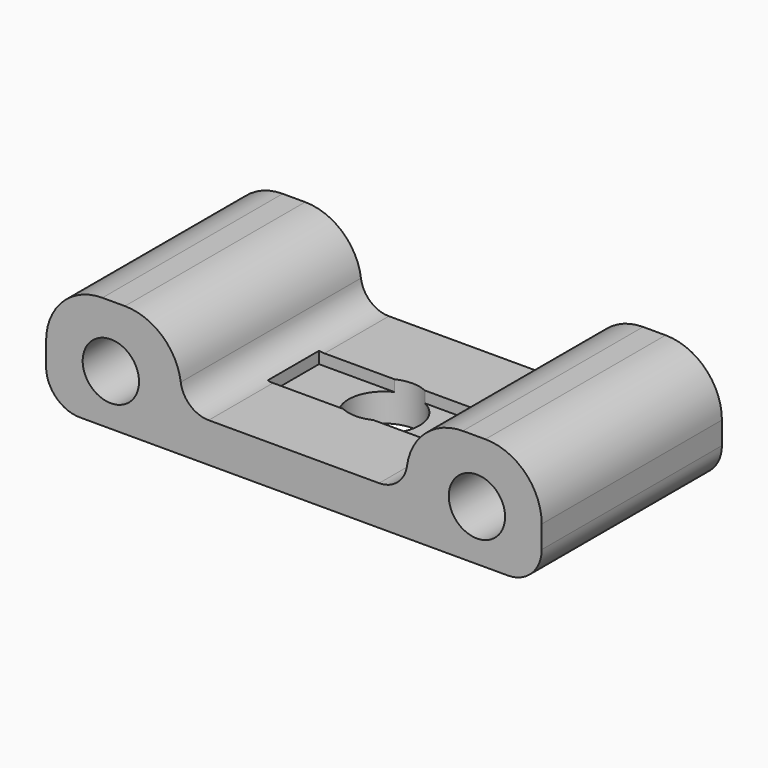
from build123d import *

# Parameters (mm, degrees)
F0_W          = 36
F0_H          = 20
F1_DEPTH      = 3.5
F3_DEPTH      = 1
F4_W          = 4
F4_H          = 20
F4_W_2        = 8
F5_DEPTH      = 10
F6_R          = 2.5
F7_DEPTH      = 20.001
F8_R          = 5
F9_R          = 3
F10_T4_DEPTH  = 20
F10_T10_DEPTH = 20
F10_T16_DEPTH = 20
F10_T23_DEPTH = 20
F10_T29_DEPTH = 20
F10_T35_DEPTH = 20
F10_T41_DEPTH = 20
F10_T47_DEPTH = 20
F10_T54_DEPTH = 20
F10_T60_DEPTH = 20


# Not quite as in the source:
# - a fillet or chamfer that OpenCascade refuses, or shapes differently, is made with other operations: its cross-section is extruded or revolved along the edge and cut away or added


with BuildPart() as f1:
    # F0 (on Top) → F1 (new body)
    with BuildSketch(Plane.XY):
        Rectangle(F0_W, F0_H)
        with BuildLine():
            ThreePointArc((3.15, 0), (0, -3.15), (-3.15, 0))
            ThreePointArc((-3.15, 0), (0, 3.15), (3.15, 0))
        make_face(mode=Mode.SUBTRACT)
    extrude(amount=F1_DEPTH)

    # F2 (on face) → F3 (cut)
    with BuildSketch(Plane.XY.offset(3.5)):
        with BuildLine():
            Line((-1.3416407865, 2.85), (-8.05, 2.85))
            Line((-8.05, 2.85), (-8.05, -2.85))
            Line((-8.05, -2.85), (-1.3416407865, -2.85))
            ThreePointArc((-1.3416407865, -2.85), (-3.15, 0), (-1.3416407865, 2.85))
        make_face()
        with BuildLine():
            Line((1.3416407865, 2.85), (-1.3416407865, 2.85))
            ThreePointArc((-1.3416407865, 2.85), (-3.15, 0), (-1.3416407865, -2.85))
            Line((-1.3416407865, -2.85), (1.3416407865, -2.85))
            ThreePointArc((1.3416407865, -2.85), (2.6597620643, -1.6876509595), (3.15, 0))
            ThreePointArc((3.15, 0), (2.6597620643, 1.6876509595), (1.3416407865, 2.85))
        make_face()
        with BuildLine():
            Line((8.05, 2.85), (1.3416407865, 2.85))
            ThreePointArc((1.3416407865, 2.85), (2.6597620643, 1.6876509595), (3.15, 0))
            ThreePointArc((3.15, 0), (2.6597620643, -1.6876509595), (1.3416407865, -2.85))
            Line((1.3416407865, -2.85), (8.05, -2.85))
            Line((8.05, -2.85), (8.05, 2.85))
        make_face()
    extrude(amount=-F3_DEPTH, mode=Mode.SUBTRACT)

    # F4 (on Top) → F5 (join)
    with BuildSketch(Plane.XY):
        with Locations((20, 0)):
            Rectangle(F4_W, F4_H)
        with Locations((14, 0)):
            Rectangle(F4_W_2, F4_H)
        with Locations((-14, 0)):
            Rectangle(F4_W_2, F4_H)
        with Locations((-20, 0)):
            Rectangle(F4_W, F4_H)
    extrude(amount=F5_DEPTH)

    # F6 (on face) → F7 (cut, through all)
    with BuildSketch(Plane.XZ.offset(10)):
        with Locations((-16.25, 4.5)):
            Circle(F6_R)
        with BuildLine():
            ThreePointArc((18.75, 4.5), (16.25, 7), (13.75, 4.5))
            ThreePointArc((13.75, 4.5), (16.25, 2), (18.75, 4.5))
        make_face()
    extrude(amount=-F7_DEPTH, mode=Mode.SUBTRACT)

    # F8
    f8_edges = [f1.edges().sort_by_distance(p)[0] for p in [
        (-22, 0, 10),
        (-10, 0, 10),
        (10, 0, 10),
        (22, 0, 10),
    ]]
    fillet(f8_edges, radius=F8_R)

    # F9
    f9_edges = [f1.edges().sort_by_distance(p)[0] for p in [
        (-22, 0, 0),
        (22, 0, 0),
    ]]
    fillet(f9_edges, radius=F9_R)

    # F10: fillet of radius 2.5 on 2 edges, made by hand


with BuildPart() as f10_tool2:
    # F10_s3 → F10_t4 (new body)
    with BuildSketch(Plane.XZ.offset(10)):
        with BuildLine():
            ThreePointArc((10.0446437509, 5.6666666667), (9.2126670979, 4.1180683682), (7.5669656263, 3.5))
            Line((7.5669656263, 3.5), (7.5669656263, 3.25))
            Line((7.5669656263, 3.25), (10, 3.25))
            Line((10, 3.25), (10.25, 3.5))
            ThreePointArc((10.25, 3.5), (10.25, 5), (10.2924115633, 5.6333333333))
            Line((10.2924115633, 5.6333333333), (10.0446437509, 5.6666666667))
        make_face()
    extrude(amount=-F10_T4_DEPTH)

    split(bisect_by=Plane.YZ.offset(8.05), keep=Keep.TOP)

    split(bisect_by=Plane.XZ.offset(2.85), keep=Keep.TOP)


with BuildPart() as f1_1:
    add(f1.part)

    # F10_t1: union F10_tool2
    add(f10_tool2.part)


with BuildPart() as f10_tool8:
    # F10_s9 → F10_t10 (new body)
    with BuildSketch(Plane.XZ.offset(10)):
        with BuildLine():
            ThreePointArc((10.0446437509, 5.6666666667), (9.2126670979, 4.1180683682), (7.5669656263, 3.5))
            Line((7.5669656263, 3.5), (7.5669656263, 3.25))
            Line((7.5669656263, 3.25), (10, 3.25))
            Line((10, 3.25), (10.25, 3.5))
            ThreePointArc((10.25, 3.5), (10.25, 5), (10.2924115633, 5.6333333333))
            Line((10.2924115633, 5.6333333333), (10.0446437509, 5.6666666667))
        make_face()
    extrude(amount=-F10_T10_DEPTH)

    split(bisect_by=Plane.YZ.offset(8.05), keep=Keep.BOTTOM)

    split(bisect_by=Plane.XZ.offset(2.85), keep=Keep.TOP)


with BuildPart() as f1_2:
    add(f1_1.part)

    # F10_t7: union F10_tool8
    add(f10_tool8.part)


with BuildPart() as f10_tool14:
    # F10_s15 → F10_t16 (new body)
    with BuildSketch(Plane.XZ.offset(10)):
        with BuildLine():
            ThreePointArc((10.0446437509, 5.6666666667), (9.2126670979, 4.1180683682), (7.5669656263, 3.5))
            Line((7.5669656263, 3.5), (7.5669656263, 3.25))
            Line((7.5669656263, 3.25), (10, 3.25))
            Line((10, 3.25), (10.25, 3.5))
            ThreePointArc((10.25, 3.5), (10.25, 5), (10.2924115633, 5.6333333333))
            Line((10.2924115633, 5.6333333333), (10.0446437509, 5.6666666667))
        make_face()
    extrude(amount=-F10_T16_DEPTH)

    split(bisect_by=Plane.XZ.offset(-2.85), keep=Keep.TOP)

    split(bisect_by=Plane.YZ.offset(8.05), keep=Keep.TOP)

    split(bisect_by=Plane.XZ.offset(2.85), keep=Keep.BOTTOM)


with BuildPart() as f1_3:
    add(f1_2.part)

    # F10_t13: union F10_tool14
    add(f10_tool14.part)


with BuildPart() as f10_tool21:
    # F10_s22 → F10_t23 (new body)
    with BuildSketch(Plane.XZ.offset(10)):
        with BuildLine():
            ThreePointArc((10.0446437509, 5.6666666667), (9.2126670979, 4.1180683682), (7.5669656263, 3.5))
            Line((7.5669656263, 3.5), (7.5669656263, 3.25))
            Line((7.5669656263, 3.25), (10, 3.25))
            Line((10, 3.25), (10.25, 3.5))
            ThreePointArc((10.25, 3.5), (10.25, 5), (10.2924115633, 5.6333333333))
            Line((10.2924115633, 5.6333333333), (10.0446437509, 5.6666666667))
        make_face()
    extrude(amount=-F10_T23_DEPTH)

    split(bisect_by=Plane.XZ.offset(-2.85), keep=Keep.BOTTOM)

    split(bisect_by=Plane.YZ.offset(8.05), keep=Keep.TOP)


with BuildPart() as f1_4:
    add(f1_3.part)

    # F10_t20: union F10_tool21
    add(f10_tool21.part)


with BuildPart() as f10_tool27:
    # F10_s28 → F10_t29 (new body)
    with BuildSketch(Plane.XZ.offset(10)):
        with BuildLine():
            ThreePointArc((10.0446437509, 5.6666666667), (9.2126670979, 4.1180683682), (7.5669656263, 3.5))
            Line((7.5669656263, 3.5), (7.5669656263, 3.25))
            Line((7.5669656263, 3.25), (10, 3.25))
            Line((10, 3.25), (10.25, 3.5))
            ThreePointArc((10.25, 3.5), (10.25, 5), (10.2924115633, 5.6333333333))
            Line((10.2924115633, 5.6333333333), (10.0446437509, 5.6666666667))
        make_face()
    extrude(amount=-F10_T29_DEPTH)

    split(bisect_by=Plane.XZ.offset(-2.85), keep=Keep.BOTTOM)

    split(bisect_by=Plane.YZ.offset(8.05), keep=Keep.BOTTOM)


with BuildPart() as f1_5:
    add(f1_4.part)

    # F10_t26: union F10_tool27
    add(f10_tool27.part)


with BuildPart() as f10_tool33:
    # F10_s34 → F10_t35 (new body)
    with BuildSketch(Plane.XZ.offset(-10)):
        with BuildLine():
            ThreePointArc((-7.5669656263, 3.5), (-9.2126670979, 4.1180683682), (-10.0446437509, 5.6666666667))
            Line((-10.0446437509, 5.6666666667), (-10.2924115633, 5.6333333333))
            ThreePointArc((-10.2924115633, 5.6333333333), (-10.25, 5), (-10.25, 3.5))
            Line((-10.25, 3.5), (-10, 3.25))
            Line((-10, 3.25), (-7.5669656263, 3.25))
            Line((-7.5669656263, 3.25), (-7.5669656263, 3.5))
        make_face()
    extrude(amount=F10_T35_DEPTH)

    split(bisect_by=Plane.XZ.offset(-2.85), keep=Keep.BOTTOM)

    split(bisect_by=Plane.YZ.offset(-8.05), keep=Keep.TOP)


with BuildPart() as f1_6:
    add(f1_5.part)

    # F10_t32: union F10_tool33
    add(f10_tool33.part)


with BuildPart() as f10_tool39:
    # F10_s40 → F10_t41 (new body)
    with BuildSketch(Plane.XZ.offset(-10)):
        with BuildLine():
            ThreePointArc((-7.5669656263, 3.5), (-9.2126670979, 4.1180683682), (-10.0446437509, 5.6666666667))
            Line((-10.0446437509, 5.6666666667), (-10.2924115633, 5.6333333333))
            ThreePointArc((-10.2924115633, 5.6333333333), (-10.25, 5), (-10.25, 3.5))
            Line((-10.25, 3.5), (-10, 3.25))
            Line((-10, 3.25), (-7.5669656263, 3.25))
            Line((-7.5669656263, 3.25), (-7.5669656263, 3.5))
        make_face()
    extrude(amount=F10_T41_DEPTH)

    split(bisect_by=Plane.XZ.offset(-2.85), keep=Keep.BOTTOM)

    split(bisect_by=Plane.YZ.offset(-8.05), keep=Keep.BOTTOM)


with BuildPart() as f1_7:
    add(f1_6.part)

    # F10_t38: union F10_tool39
    add(f10_tool39.part)


with BuildPart() as f10_tool45:
    # F10_s46 → F10_t47 (new body)
    with BuildSketch(Plane.XZ.offset(-10)):
        with BuildLine():
            ThreePointArc((-7.5669656263, 3.5), (-9.2126670979, 4.1180683682), (-10.0446437509, 5.6666666667))
            Line((-10.0446437509, 5.6666666667), (-10.2924115633, 5.6333333333))
            ThreePointArc((-10.2924115633, 5.6333333333), (-10.25, 5), (-10.25, 3.5))
            Line((-10.25, 3.5), (-10, 3.25))
            Line((-10, 3.25), (-7.5669656263, 3.25))
            Line((-7.5669656263, 3.25), (-7.5669656263, 3.5))
        make_face()
    extrude(amount=F10_T47_DEPTH)

    split(bisect_by=Plane.XZ.offset(-2.85), keep=Keep.TOP)

    split(bisect_by=Plane.YZ.offset(-8.05), keep=Keep.BOTTOM)

    split(bisect_by=Plane.XZ.offset(2.85), keep=Keep.BOTTOM)


with BuildPart() as f1_8:
    add(f1_7.part)

    # F10_t44: union F10_tool45
    add(f10_tool45.part)


with BuildPart() as f10_tool52:
    # F10_s53 → F10_t54 (new body)
    with BuildSketch(Plane.XZ.offset(-10)):
        with BuildLine():
            ThreePointArc((-7.5669656263, 3.5), (-9.2126670979, 4.1180683682), (-10.0446437509, 5.6666666667))
            Line((-10.0446437509, 5.6666666667), (-10.2924115633, 5.6333333333))
            ThreePointArc((-10.2924115633, 5.6333333333), (-10.25, 5), (-10.25, 3.5))
            Line((-10.25, 3.5), (-10, 3.25))
            Line((-10, 3.25), (-7.5669656263, 3.25))
            Line((-7.5669656263, 3.25), (-7.5669656263, 3.5))
        make_face()
    extrude(amount=F10_T54_DEPTH)

    split(bisect_by=Plane.YZ.offset(-8.05), keep=Keep.TOP)

    split(bisect_by=Plane.XZ.offset(2.85), keep=Keep.TOP)


with BuildPart() as f1_9:
    add(f1_8.part)

    # F10_t51: union F10_tool52
    add(f10_tool52.part)


with BuildPart() as f10_tool58:
    # F10_s59 → F10_t60 (new body)
    with BuildSketch(Plane.XZ.offset(-10)):
        with BuildLine():
            ThreePointArc((-7.5669656263, 3.5), (-9.2126670979, 4.1180683682), (-10.0446437509, 5.6666666667))
            Line((-10.0446437509, 5.6666666667), (-10.2924115633, 5.6333333333))
            ThreePointArc((-10.2924115633, 5.6333333333), (-10.25, 5), (-10.25, 3.5))
            Line((-10.25, 3.5), (-10, 3.25))
            Line((-10, 3.25), (-7.5669656263, 3.25))
            Line((-7.5669656263, 3.25), (-7.5669656263, 3.5))
        make_face()
    extrude(amount=F10_T60_DEPTH)

    split(bisect_by=Plane.YZ.offset(-8.05), keep=Keep.BOTTOM)

    split(bisect_by=Plane.XZ.offset(2.85), keep=Keep.TOP)


with BuildPart() as f1_10:
    add(f1_9.part)

    # F10_t57: union F10_tool58
    add(f10_tool58.part)


solid = f1_10.part
